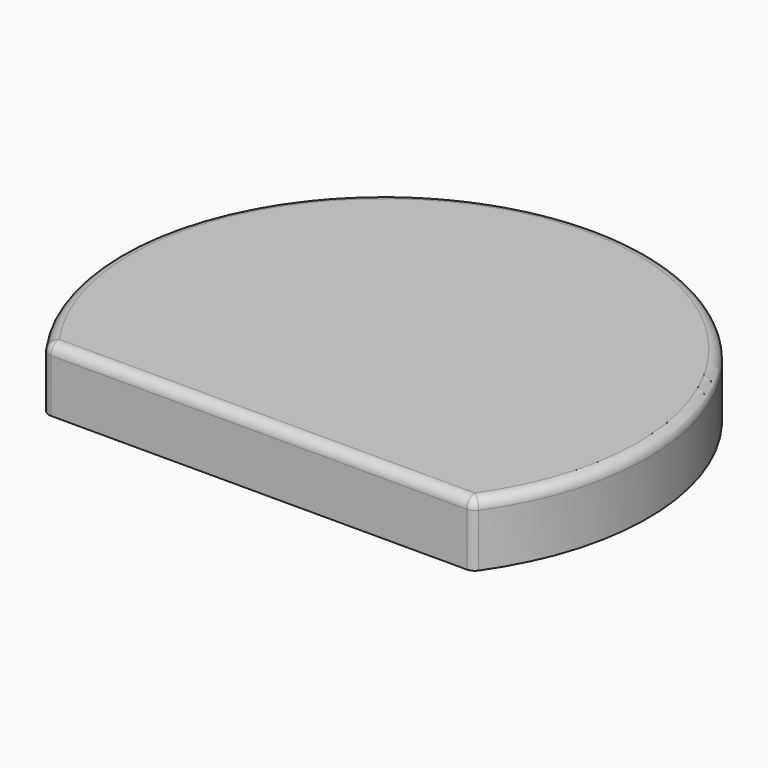
from build123d import *

# Parameters (mm, degrees)
F1_DEPTH = 6.2
F2_R     = 1


with BuildPart() as f1:
    # F0 (on Top) → F1 (new body)
    with BuildSketch(Plane.XY):
        with BuildLine():
            ThreePointArc((20.897846779, -15.3), (0, 25.9), (-20.897846779, -15.3))
            Line((-20.897846779, -15.3), (20.897846779, -15.3))
        make_face()
    extrude(amount=F1_DEPTH)

    # F2
    f2_edges = [f1.edges().sort_by_distance(p)[0] for p in [
        (-20.897847, -15.3, 3.1),
        (0, 25.9, 6.2),
        (0, -15.3, 6.2),
        (20.897847, -15.3, 3.1),
    ]]
    fillet(f2_edges, radius=F2_R)


solid = f1.part
